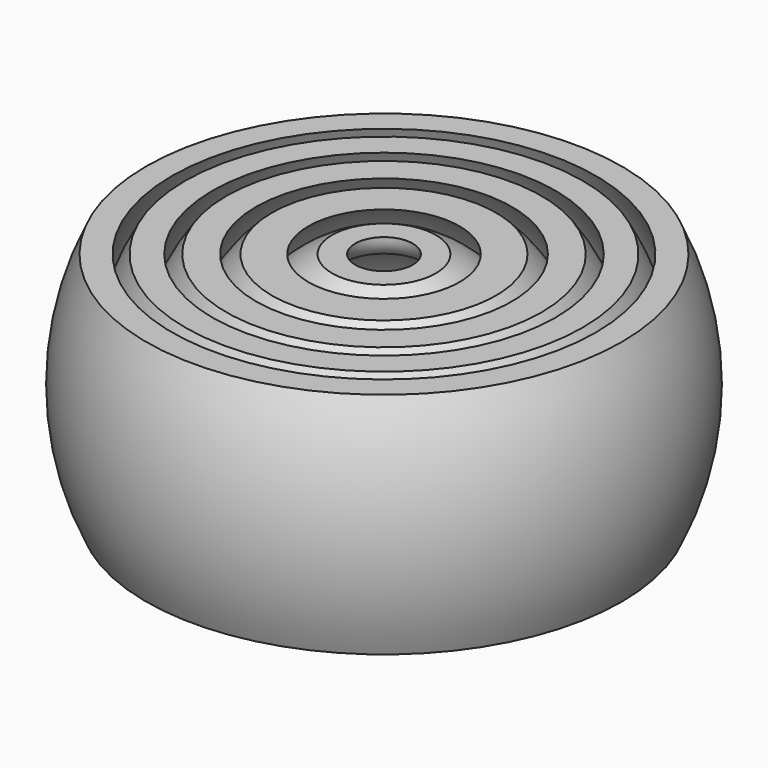
from build123d import *

# Parameters (mm, degrees)
F3_T = -1.6


# Not quite as in the source:
# - a fillet or chamfer that OpenCascade refuses, or shapes differently, is made with other operations: its cross-section is extruded or revolved along the edge and cut away or added


with BuildPart() as f2:
    # F1 (on Front) → F2 (revolve)
    with BuildSketch(Plane.XZ):
        with BuildLine():
            Line((-2, 7.9332899209), (-3.6, 7.9332899209))
            ThreePointArc((-3.6, 7.9332899209), (-7.098863782, 5.050071482), (-8.6751621405, 0.799156308))
            ThreePointArc((-8.6751621405, 0.799156308), (-8.1333673406, 0.5525463258), (-7.9118935352, 0))
            ThreePointArc((-7.9118935352, 0), (-8.1333673406, -0.5525463258), (-8.6751621405, -0.799156308))
            ThreePointArc((-8.6751621405, -0.799156308), (-7.098863782, -5.050071482), (-3.6, -7.9332899209))
            Line((-3.6, -7.9332899209), (-2, -7.9332899209))
            Line((-2, -7.9332899209), (-2, 0))
            Line((-2, 0), (-2, 7.9332899209))
        make_face()
    revolve(axis=Axis((0, 0, -1.2736130784), (0, 0, -1)))

    # F3
    f3_openings = [f2.faces().sort_by_distance(p)[0] for p in [
        (2, 0, 0),
    ]]
    offset(amount=F3_T, openings=f3_openings)

    # F4: fillet of radius 1.6 on 2 edges, made by hand

    # F4_s1 → F4_t2 (revolve, cut)
    with BuildSketch(Plane.XZ):
        with BuildLine():
            ThreePointArc((-2, -7.8912182479), (-2.346365688, -6.8970346573), (-3.2355012647, -6.3332899209))
            Line((-3.2355012647, -6.3332899209), (-3.22821129, -6.3021313544))
            ThreePointArc((-3.22821129, -6.3021313544), (-2.6177506324, -6.3012899209), (-2, -6.3012899209))
            Line((-2, -6.3012899209), (-1.968, -6.3332899209))
            Line((-1.968, -6.3332899209), (-1.968, -7.8912182479))
            Line((-1.968, -7.8912182479), (-2, -7.8912182479))
        make_face()
    revolve(axis=Axis((0, 0, -6.3332899209), (0, 0, -1)), mode=Mode.SUBTRACT)

    # F4_s3 → F4_t4 (revolve, cut)
    with BuildSketch(Plane.XZ):
        with BuildLine():
            ThreePointArc((-2, 7.8912182479), (-2.346365688, 6.8970346573), (-3.2355012647, 6.3332899209))
            Line((-3.2355012647, 6.3332899209), (-3.22821129, 6.3021313544))
            ThreePointArc((-3.22821129, 6.3021313544), (-2.6177506324, 6.3012899209), (-2, 6.3012899209))
            Line((-2, 6.3012899209), (-1.968, 6.3332899209))
            Line((-1.968, 6.3332899209), (-1.968, 7.8912182479))
            Line((-1.968, 7.8912182479), (-2, 7.8912182479))
        make_face()
    revolve(axis=Axis((0, 0, 6.3332899209), (0, 0, -1)), mode=Mode.SUBTRACT)


with BuildPart() as f2b:
    # F1 (on Front) → F2, piece 2 (revolve)
    with BuildSketch(Plane.XZ):
        with BuildLine():
            ThreePointArc((-9.5118935352, 0), (-8.3783140756, 4.5033289771), (-5.2477642531, 7.9332899209))
            Line((-5.2477642531, 7.9332899209), (-7.780558397, 7.9332899209))
            ThreePointArc((-7.780558397, 7.9332899209), (-10.0837575244, 4.6681915264), (-11.0830955631, 0.799481505))
            ThreePointArc((-11.0830955631, 0.799481505), (-10.5361165047, 0.5554104889), (-10.3118935352, 0))
            ThreePointArc((-10.3118935352, 0), (-10.5361165047, -0.5554104889), (-11.0830955631, -0.799481505))
            ThreePointArc((-11.0830955631, -0.799481505), (-10.0837575244, -4.6681915264), (-7.780558397, -7.9332899209))
            Line((-7.780558397, -7.9332899209), (-5.2477642531, -7.9332899209))
            ThreePointArc((-5.2477642531, -7.9332899209), (-8.3783140756, -4.5033289771), (-9.5118935352, 0))
        make_face()
    revolve(axis=Axis((0, 0, -1.2736130784), (0, 0, -1)))


with BuildPart() as f2c:
    # F1 (on Front) → F2, piece 3 (revolve)
    with BuildSketch(Plane.XZ):
        with BuildLine():
            ThreePointArc((-11.9118935352, 1.99e-08), (-11.1296681043, 4.2454323082), (-8.8857255542, 7.9332899209))
            Line((-8.8857255542, 7.9332899209), (-10.9377409888, 7.9332899209))
            ThreePointArc((-10.9377409888, 7.9332899209), (-12.723167286, 4.5488769074), (-13.4882106962, 0.7996493751))
            ThreePointArc((-13.4882106962, 0.7996493751), (-12.9378960303, 0.5572493736), (-12.7118935352, 0))
            ThreePointArc((-12.7118935352, 0), (-12.9378960303, -0.5572493736), (-13.4882106962, -0.7996493751))
            ThreePointArc((-13.4882106962, -0.7996493751), (-12.723167286, -4.5488769074), (-10.9377409888, -7.9332899209))
            Line((-10.9377409888, -7.9332899209), (-8.8857255542, -7.9332899209))
            ThreePointArc((-8.8857255542, -7.9332899209), (-11.1296681114, -4.2454322896), (-11.9118935352, 1.99e-08))
        make_face()
    revolve(axis=Axis((0, 0, -1.2736130784), (0, 0, -1)))


with BuildPart() as f2d:
    # F1 (on Front) → F2, piece 4 (revolve)
    with BuildSketch(Plane.XZ):
        with BuildLine():
            ThreePointArc((-14.3118935352, 0), (-13.6987599556, 4.1441853533), (-11.9118935352, 7.9332899209))
            Line((-11.9118935352, 7.9332899209), (-13.7931601494, 7.9332899209))
            ThreePointArc((-13.7931601494, 7.9332899209), (-15.2650194025, 4.4908282663), (-15.8917827923, 0.7997471838))
            ThreePointArc((-15.8917827923, 0.7997471838), (-15.3391420209, 0.558529948), (-15.1118935352, 0))
            ThreePointArc((-15.1118935352, 0), (-15.3391420209, -0.558529948), (-15.8917827923, -0.7997471838))
            ThreePointArc((-15.8917827923, -0.7997471838), (-15.2650194025, -4.4908282663), (-13.7931601494, -7.9332899209))
            Line((-13.7931601494, -7.9332899209), (-11.9118935352, -7.9332899209))
            ThreePointArc((-11.9118935352, -7.9332899209), (-13.6987599556, -4.1441853533), (-14.3118935352, 0))
        make_face()
    revolve(axis=Axis((0, 0, -1.2736130784), (0, 0, -1)))


with BuildPart() as f2e:
    # F1 (on Front) → F2, piece 5 (revolve)
    with BuildSketch(Plane.XZ):
        with BuildLine():
            ThreePointArc((-16.7118935352, 0), (-16.2033968167, 4.0911266336), (-14.70885096, 7.9332899209))
            Line((-14.70885096, 7.9332899209), (-16.5041920698, 7.9332899209))
            ThreePointArc((-16.5041920698, 7.9332899209), (-18.3118935352, 0), (-16.5041920698, -7.9332899209))
            Line((-16.5041920698, -7.9332899209), (-14.70885096, -7.9332899209))
            ThreePointArc((-14.70885096, -7.9332899209), (-16.2033968167, -4.0911266336), (-16.7118935352, 0))
        make_face()
    revolve(axis=Axis((0, 0, -1.2736130784), (0, 0, -1)))


solid = Compound([f2.part, f2b.part, f2c.part, f2d.part, f2e.part])
